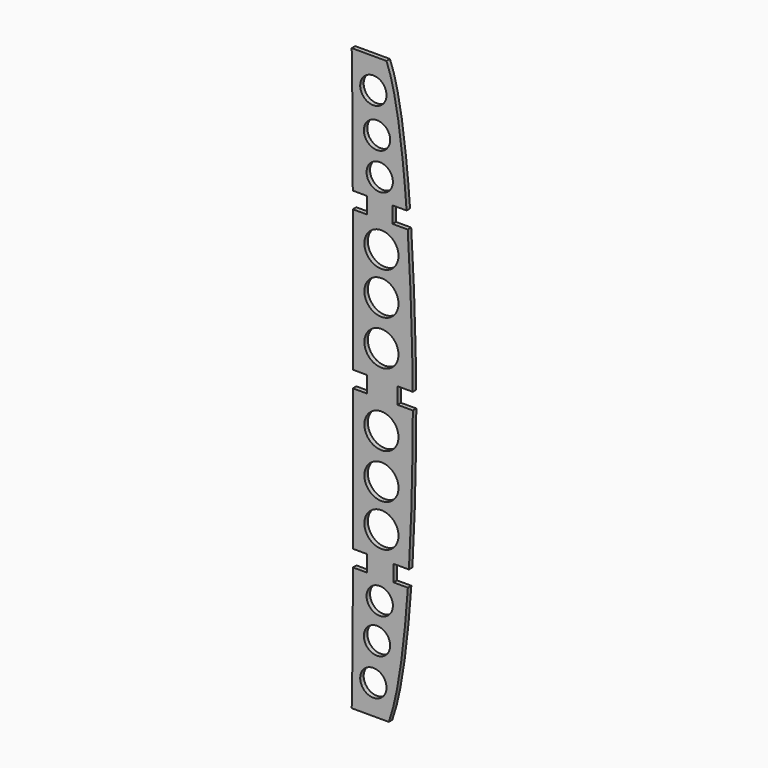
from build123d import *

# Parameters (mm, degrees)
F0_R     = 15.6427266016
F0_R_2   = 12.0636627394
F1_DEPTH = 4


# Not quite as in the source:
# - a feature names something its author has since deleted; it is built from what else it names


with BuildPart() as f1:
    # F0 (on Front) → F1 (new body)
    with BuildSketch(Plane.XZ):
        with BuildLine():
            add(Edge.make_bspline(
                [(606.664408162, -6.3581708061), (610.2484126071, -61.6736918338), (611.0695149221, -116.339928141), (611.2557314215, -135.8581708061)],
                knots=[116.1389128405, 116.1389128405, 116.1389128405, 116.1389128405, 238.5747877883, 238.5747877883, 238.5747877883, 238.5747877883], degree=3))
            Line((606.664408162, -6.3581708061), (592.664408162, -6.3581708061))
            Line((592.664408162, -6.3581708061), (592.664408162, 1.1418291939))
            Line((592.664408162, 1.1418291939), (569.3247318268, 1.1418291939))
            Line((569.3247318268, 1.1418291939), (569.3247318268, -6.3581708061))
            Line((569.3247318268, -6.3581708061), (556.3105202547, -6.3581708061))
            add(Edge.make_bspline(
                [(556.3105202547, -6.3581708062), (556.3560675182, -46.8595634464), (556.3040983749, -91.0874507126), (556.321195241, -135.8581708062)],
                knots=[0.2731602209, 0.2731602209, 0.2731602209, 0.2731602209, 0.4883298337, 0.4883298337, 0.4883298337, 0.4883298337], degree=3))
            Line((556.321195241, -135.8581708061), (569.3247318268, -135.8581708061))
            Line((569.3247318268, -135.8581708061), (569.3247318268, -143.3581708061))
            Line((569.3247318268, -143.3581708061), (597.3095011307, -143.3581708061))
            Line((597.3095011307, -143.3581708061), (597.3095011307, -135.8581708061))
            Line((597.3095011307, -135.8581708061), (611.2557314215, -135.8581708061))
        make_face()
        with Locations((582.5758576393, -110.06578058)):
            Circle(F0_R, mode=Mode.SUBTRACT)
        with Locations((582.5758576393, -69.0548494458)):
            Circle(F0_R, mode=Mode.SUBTRACT)
        with Locations((582.5758576393, -30.3874015808)):
            Circle(F0_R, mode=Mode.SUBTRACT)
        with BuildLine():
            add(Edge.make_bspline(
                [(587.1910579171, 123.3613954191), (596.407592129, 101.4742246466), (602.1031854422, 55.9678384662), (605.6225226157, 8.6418291939)],
                knots=[0, 0, 0, 0, 105.0647905127, 105.0647905127, 105.0647905127, 105.0647905127], degree=3))
            Line((587.1910579171, 123.3613954191), (563.1910579171, 123.3613954191))
            Line((563.1910579171, 123.3613954191), (555.3247318268, 123.3613954191))
            add(Edge.make_bspline(
                [(555.3247318268, 123.3613954191), (555.9675431408, 93.7069693731), (556.2055580917, 53.8758795815), (556.2885566673, 8.6418291939)],
                knots=[0, 0, 0, 0, 0.2462769496, 0.2462769496, 0.2462769496, 0.2462769496], degree=3))
            Line((556.2885566673, 8.6418291939), (569.3247318268, 8.6418291939))
            Line((569.3247318268, 8.6418291939), (569.3247318268, 1.1418291939))
            Line((569.3247318268, 1.1418291939), (592.664408162, 1.1418291939))
            Line((592.664408162, 1.1418291939), (592.664408162, 8.6418291939))
            Line((592.664408162, 8.6418291939), (605.6225226157, 8.6418291939))
        make_face()
        with Locations((581.0006856918, 27.6772994548)):
            Circle(F0_R_2, mode=Mode.SUBTRACT)
        with Locations((575.1569867134, 95.7145318389)):
            Circle(F0_R_2, mode=Mode.SUBTRACT)
        with Locations((578.4962773323, 60.652397573)):
            Circle(F0_R_2, mode=Mode.SUBTRACT)
        with BuildLine():
            add(Edge.make_bspline(
                [(607.7513419726, -280.3581708061), (611.0463615473, -224.7368336409), (611.3157540895, -170.3281819541), (611.3171415076, -150.8581708061)],
                knots=[112.8825860344, 112.8825860344, 112.8825860344, 112.8825860344, 237.6045572103, 237.6045572103, 237.6045572103, 237.6045572103], degree=3))
            Line((611.3171415076, -150.8581708061), (611.3095011307, -150.8581708061))
            Line((611.3095011307, -150.8581708061), (597.3095011307, -150.8581708061))
            Line((597.3095011307, -150.8581708061), (597.3095011307, -143.3581708061))
            Line((597.3095011307, -143.3581708061), (569.3247318268, -143.3581708061))
            Line((569.3247318268, -143.3581708061), (569.3247318268, -150.8581708061))
            Line((569.3247318268, -150.8581708061), (556.3296648649, -150.8581708061))
            add(Edge.make_bspline(
                [(556.3296648649, -150.8581708062), (556.3627723501, -195.2400977423), (556.4619608218, -239.7521985209), (556.4380859402, -280.3581708061)],
                knots=[0.5123348883, 0.5123348883, 0.5123348883, 0.5123348883, 0.7252628697, 0.7252628697, 0.7252628697, 0.7252628697], degree=3))
            Line((556.4380859402, -280.3581708061), (569.3247318268, -280.3581708061))
            Line((569.3247318268, -280.3581708061), (569.3247318268, -287.8581708061))
            Line((569.3247318268, -287.8581708061), (569.3247318268, -295.3581708061))
            Line((569.3247318268, -295.3581708061), (556.4230475774, -295.3581708061))
            add(Edge.make_bspline(
                [(556.4230475774, -295.3581708061), (556.3560187283, -341.4793760002), (556.0897539461, -381.6099515969), (555.3247318268, -409.3581708061)],
                knots=[0.7518138312, 0.7518138312, 0.7518138312, 0.7518138312, 1, 1, 1, 1], degree=3))
            Line((555.3247318268, -409.3581708061), (556.8649172783, -409.3581708061))
            Line((556.8649172783, -409.3581708061), (589.3247318268, -409.3581708061))
            add(Edge.make_bspline(
                [(589.3247318268, -409.3581708061), (598.3171301483, -384.7473411865), (603.6401377777, -340.6568702112), (606.7877271908, -295.3581708061)],
                knots=[0, 0, 0, 0, 101.6745497642, 101.6745497642, 101.6745497642, 101.6745497642], degree=3))
            Line((606.7877271908, -295.3581708061), (605.6225226157, -295.3581708061))
            Line((605.6225226157, -295.3581708061), (593.664408162, -295.3581708061))
            Line((593.664408162, -295.3581708061), (593.664408162, -280.3581708061))
            Line((593.664408162, -280.3581708061), (606.664408162, -280.3581708061))
            Line((606.664408162, -280.3581708061), (607.7513419726, -280.3581708061))
        make_face()
        with Locations((575.1569867134, -382.4308734512)):
            Circle(F0_R_2, mode=Mode.SUBTRACT)
        with Locations((578.4962773323, -347.3687391853)):
            Circle(F0_R_2, mode=Mode.SUBTRACT)
        with Locations((581.0006856918, -314.3936410671)):
            Circle(F0_R_2, mode=Mode.SUBTRACT)
        with Locations((582.5758576393, -256.3289400315)):
            Circle(F0_R, mode=Mode.SUBTRACT)
        with Locations((582.5758576393, -217.6614921665)):
            Circle(F0_R, mode=Mode.SUBTRACT)
        with Locations((582.5758576393, -176.6505610322)):
            Circle(F0_R, mode=Mode.SUBTRACT)
    extrude(amount=F1_DEPTH)


solid = f1.part
